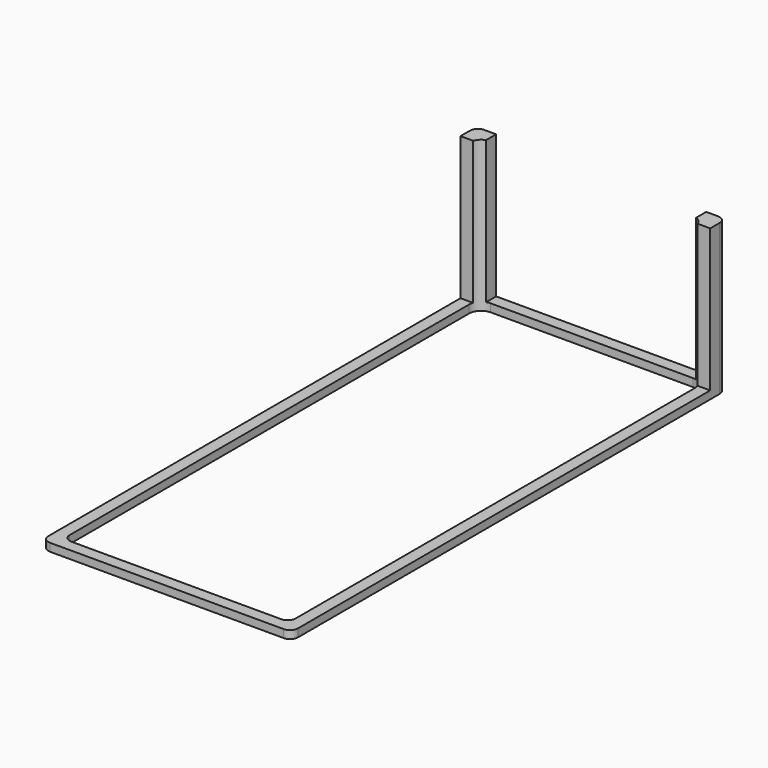
from build123d import *

# Parameters (mm, degrees)
F0_W         = 63
F0_H         = 137
F0_W_2       = 57
F0_H_2       = 131
F1_DEPTH     = 2
F4_DEPTH     = 36
F5_T4_DEPTH  = 38
F5_T10_DEPTH = 38
F5_T17_DEPTH = 38
F5_T23_DEPTH = 38
F5_T30_DEPTH = 38
F5_T36_DEPTH = 38
F5_T43_DEPTH = 38
F5_T49_DEPTH = 38
F6_R         = 2


# Not quite as in the source:
# - a fillet or chamfer that OpenCascade refuses, or shapes differently, is made with other operations: its cross-section is extruded or revolved along the edge and cut away or added


with BuildPart() as f1:
    # F0 (on Top) → F1 (new body)
    with BuildSketch(Plane.XY):
        Rectangle(F0_W, F0_H)
        Rectangle(F0_W_2, F0_H_2, mode=Mode.SUBTRACT)
    extrude(amount=F1_DEPTH)

    # F3 (on face) → F4 (join, through all)
    with BuildSketch(Plane.XY.offset(2)):
        Polygon((-26.5, 68.5), (-31.5, 68.5), (-31.5, 63.5), (-28.5, 63.5), (-28.5, 65.5), (-26.5, 65.5), align=None)
        Polygon((31.5, 68.5), (26.5, 68.5), (26.5, 65.5), (28.5, 65.5), (28.5, 63.5), (31.5, 63.5), align=None)
    extrude(amount=F4_DEPTH)

    # F5: fillet of radius 3 on 2 edges, made by hand


with BuildPart() as f5_tool2:
    # F5_s3 → F5_t4 (new body)
    with BuildSketch(Plane.XY):
        with BuildLine():
            ThreePointArc((-25.5, 65.5), (-27.6213203436, 64.6213203436), (-28.5, 62.5))
            Line((-28.5, 62.5), (-28.5, 65.5))
            Line((-28.5, 65.5), (-25.5, 65.5))
        make_face()
    extrude(amount=F5_T4_DEPTH)

    split(bisect_by=Plane.XY.offset(2), keep=Keep.BOTTOM)

    split(bisect_by=Plane.YZ.offset(-26.5), keep=Keep.TOP)


with BuildPart() as f1_1:
    add(f1.part)

    # F5_t1: union F5_tool2
    add(f5_tool2.part)


with BuildPart() as f5_tool8:
    # F5_s9 → F5_t10 (new body)
    with BuildSketch(Plane.XY):
        with BuildLine():
            ThreePointArc((-25.5, 65.5), (-27.6213203436, 64.6213203436), (-28.5, 62.5))
            Line((-28.5, 62.5), (-28.5, 65.5))
            Line((-28.5, 65.5), (-25.5, 65.5))
        make_face()
    extrude(amount=F5_T10_DEPTH)

    split(bisect_by=Plane.XY.offset(2), keep=Keep.BOTTOM)

    split(bisect_by=Plane.XZ.offset(-63.5), keep=Keep.BOTTOM)

    split(bisect_by=Plane.YZ.offset(-26.5), keep=Keep.BOTTOM)


with BuildPart() as f1_2:
    add(f1_1.part)

    # F5_t7: union F5_tool8
    add(f5_tool8.part)


with BuildPart() as f5_tool15:
    # F5_s16 → F5_t17 (new body)
    with BuildSketch(Plane.XY):
        with BuildLine():
            ThreePointArc((-25.5, 65.5), (-27.6213203436, 64.6213203436), (-28.5, 62.5))
            Line((-28.5, 62.5), (-28.5, 65.5))
            Line((-28.5, 65.5), (-25.5, 65.5))
        make_face()
    extrude(amount=F5_T17_DEPTH)

    split(bisect_by=Plane.XY.offset(2), keep=Keep.BOTTOM)

    split(bisect_by=Plane.XZ.offset(-63.5), keep=Keep.TOP)


with BuildPart() as f1_3:
    add(f1_2.part)

    # F5_t14: union F5_tool15
    add(f5_tool15.part)


with BuildPart() as f5_tool21:
    # F5_s22 → F5_t23 (new body)
    with BuildSketch(Plane.XY):
        with BuildLine():
            ThreePointArc((-25.5, 65.5), (-27.6213203436, 64.6213203436), (-28.5, 62.5))
            Line((-28.5, 62.5), (-28.5, 65.5))
            Line((-28.5, 65.5), (-25.5, 65.5))
        make_face()
    extrude(amount=F5_T23_DEPTH)

    split(bisect_by=Plane.XY.offset(2), keep=Keep.TOP)

    split(bisect_by=Plane.XZ.offset(-63.5), keep=Keep.BOTTOM)

    split(bisect_by=Plane.YZ.offset(-26.5), keep=Keep.BOTTOM)


with BuildPart() as f1_4:
    add(f1_3.part)

    # F5_t20: union F5_tool21
    add(f5_tool21.part)


with BuildPart() as f5_tool28:
    # F5_s29 → F5_t30 (new body)
    with BuildSketch(Plane.XY):
        with BuildLine():
            ThreePointArc((28.5, 62.5), (27.6213203436, 64.6213203436), (25.5, 65.5))
            Line((25.5, 65.5), (28.5, 65.5))
            Line((28.5, 65.5), (28.5, 62.5))
        make_face()
    extrude(amount=F5_T30_DEPTH)

    split(bisect_by=Plane.XY.offset(2), keep=Keep.BOTTOM)

    split(bisect_by=Plane.XZ.offset(-63.5), keep=Keep.TOP)


with BuildPart() as f1_5:
    add(f1_4.part)

    # F5_t27: union F5_tool28
    add(f5_tool28.part)


with BuildPart() as f5_tool34:
    # F5_s35 → F5_t36 (new body)
    with BuildSketch(Plane.XY):
        with BuildLine():
            ThreePointArc((28.5, 62.5), (27.6213203436, 64.6213203436), (25.5, 65.5))
            Line((25.5, 65.5), (28.5, 65.5))
            Line((28.5, 65.5), (28.5, 62.5))
        make_face()
    extrude(amount=F5_T36_DEPTH)

    split(bisect_by=Plane.XY.offset(2), keep=Keep.BOTTOM)

    split(bisect_by=Plane.XZ.offset(-63.5), keep=Keep.BOTTOM)

    split(bisect_by=Plane.YZ.offset(26.5), keep=Keep.TOP)


with BuildPart() as f1_6:
    add(f1_5.part)

    # F5_t33: union F5_tool34
    add(f5_tool34.part)


with BuildPart() as f5_tool41:
    # F5_s42 → F5_t43 (new body)
    with BuildSketch(Plane.XY):
        with BuildLine():
            ThreePointArc((28.5, 62.5), (27.6213203436, 64.6213203436), (25.5, 65.5))
            Line((25.5, 65.5), (28.5, 65.5))
            Line((28.5, 65.5), (28.5, 62.5))
        make_face()
    extrude(amount=F5_T43_DEPTH)

    split(bisect_by=Plane.XY.offset(2), keep=Keep.BOTTOM)

    split(bisect_by=Plane.YZ.offset(26.5), keep=Keep.BOTTOM)


with BuildPart() as f1_7:
    add(f1_6.part)

    # F5_t40: union F5_tool41
    add(f5_tool41.part)


with BuildPart() as f5_tool47:
    # F5_s48 → F5_t49 (new body)
    with BuildSketch(Plane.XY):
        with BuildLine():
            ThreePointArc((28.5, 62.5), (27.6213203436, 64.6213203436), (25.5, 65.5))
            Line((25.5, 65.5), (28.5, 65.5))
            Line((28.5, 65.5), (28.5, 62.5))
        make_face()
    extrude(amount=F5_T49_DEPTH)

    split(bisect_by=Plane.XY.offset(2), keep=Keep.TOP)

    split(bisect_by=Plane.XZ.offset(-63.5), keep=Keep.BOTTOM)

    split(bisect_by=Plane.YZ.offset(26.5), keep=Keep.TOP)


with BuildPart() as f1_8:
    add(f1_7.part)

    # F5_t46: union F5_tool47
    add(f5_tool47.part)

    # F6
    f6_edges = [f1_8.edges().sort_by_distance(p)[0] for p in [
        (-31.5, 68.5, 19),
        (31.5, 68.5, 19),
        (31.5, -68.5, 1),
        (-31.5, -68.5, 1),
        (28.5, -65.5, 1),
        (-28.5, -65.5, 1),
    ]]
    fillet(f6_edges, radius=F6_R)


solid = f1_8.part
